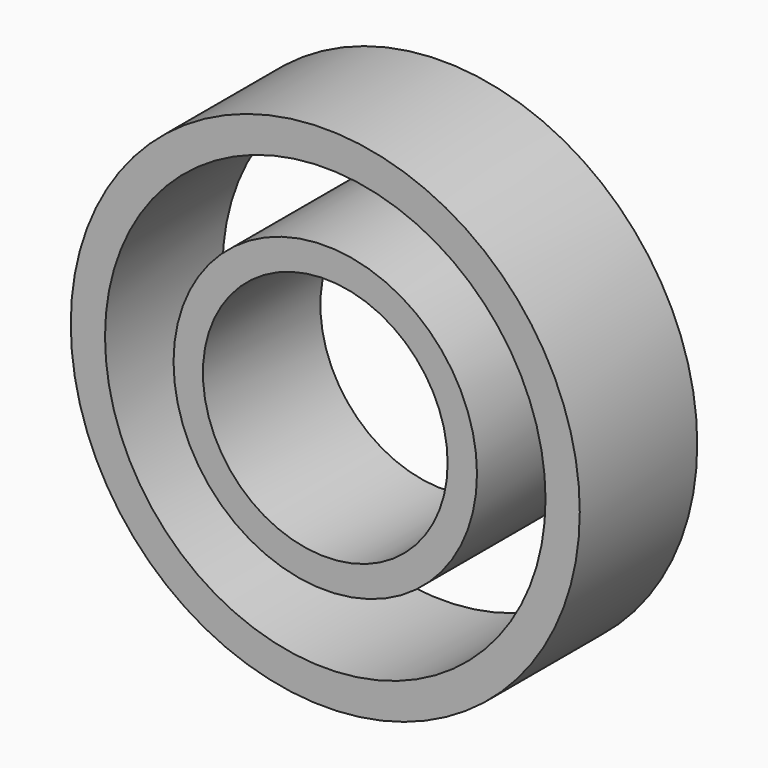
from build123d import *

# Parameters (mm, degrees)
F0_R     = 15.5
F0_R_2   = 12.5
F1_DEPTH = 15
F0_R_3   = 26
F0_R_4   = 22.5


# Not quite as in the source:
# - a feature of the source that left no trace in its solid (it failed there, or was rolled back) is left out


with BuildPart() as f1:
    # F0 (on Front) → F1 (new body)
    with BuildSketch(Plane.XZ):
        Circle(F0_R)
        Circle(F0_R_2, mode=Mode.SUBTRACT)
    extrude(amount=F1_DEPTH)


with BuildPart() as f1b:
    # F0 (on Front) → F1, piece 2 (new body)
    with BuildSketch(Plane.XZ):
        Circle(F0_R_3)
        Circle(F0_R_4, mode=Mode.SUBTRACT)
    extrude(amount=F1_DEPTH)


solid = Compound([f1.part, f1b.part])
